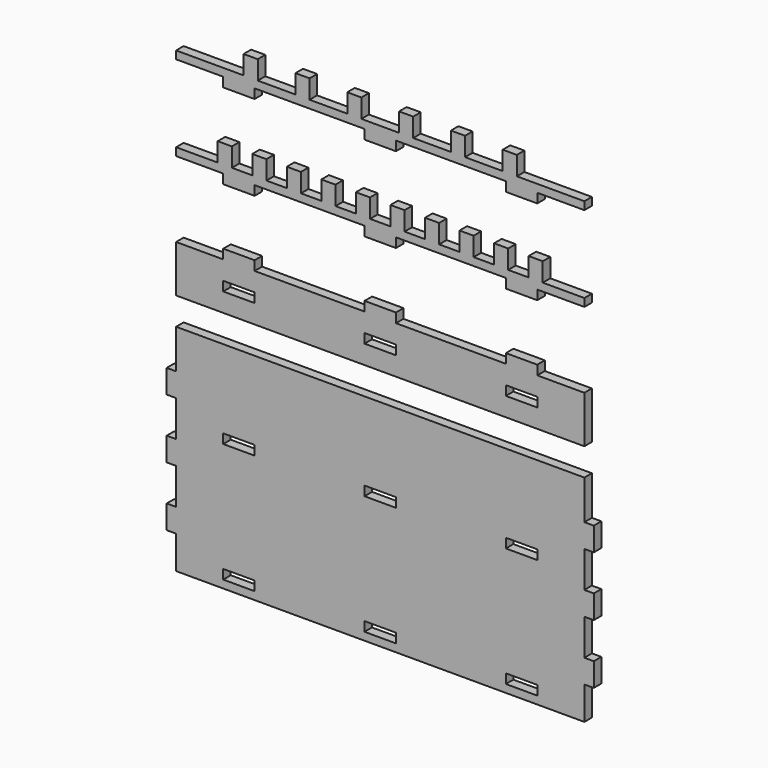
from build123d import *

# Parameters (mm, degrees)
F0_W     = 20
F0_H     = 6
F1_DEPTH = 6
F2_DEPTH = 6
F3_DEPTH = 6
F4_DEPTH = 6


# Not quite as in the source:
# - a feature names something its author has since deleted; it is built from what else it names


with BuildPart() as f1:
    # F0 (on Front) → F1 (new body)
    with BuildSketch(Plane.XZ):
        Polygon((153.699216228, -140.3053558618), (-106.300783772, -140.3053558618), (-106.300783772, -165.3053558618), (-112.300783772, -165.3053558618), (-112.300783772, -180.3053558618), (-106.300783772, -180.3053558618), (-106.300783772, -203.3053558618), (-112.300783772, -203.3053558618), (-112.300783772, -218.3053558618), (-106.300783772, -218.3053558618), (-106.300783772, -241.3053558618), (-112.300783772, -241.3053558618), (-112.300783772, -256.3053558618), (-106.300783772, -256.3053558618), (-106.300783772, -277.3053558618), (153.699216228, -277.3053558618), (153.699216228, -256.3053558618), (159.699216228, -256.3053558618), (159.699216228, -241.3053558618), (153.699216228, -241.3053558618), (153.699216228, -218.3053558618), (159.699216228, -218.3053558618), (159.699216228, -203.3053558618), (153.699216228, -203.3053558618), (153.699216228, -180.3053558618), (159.699216228, -180.3053558618), (159.699216228, -165.3053558618), (153.699216228, -165.3053558618), align=None)
        with Locations((-66.300783772, -269.3053558618)):
            Rectangle(F0_W, F0_H, mode=Mode.SUBTRACT)
        with Locations((-66.300783772, -193.3053558618)):
            Rectangle(F0_W, F0_H, mode=Mode.SUBTRACT)
        with Locations((23.699216228, -193.3053558618)):
            Rectangle(F0_W, F0_H, mode=Mode.SUBTRACT)
        with Locations((23.699216228, -269.3053558618)):
            Rectangle(F0_W, F0_H, mode=Mode.SUBTRACT)
        with Locations((113.699216228, -269.3053558618)):
            Rectangle(F0_W, F0_H, mode=Mode.SUBTRACT)
        with Locations((113.699216228, -193.3053558618)):
            Rectangle(F0_W, F0_H, mode=Mode.SUBTRACT)
    extrude(amount=F1_DEPTH)


with BuildPart() as f2:
    # F0 (on Front) → F2 (new body)
    with BuildSketch(Plane.XZ):
        Polygon((-76.300783772, -92.7685894072), (-106.300783772, -92.7685894072), (-106.300783772, -122.7685894072), (153.699216228, -122.7685894072), (153.699216228, -92.7685894072), (123.699216228, -92.7685894072), (123.699216228, -86.7685894072), (103.699216228, -86.7685894072), (103.699216228, -92.7685894072), (33.699216228, -92.7685894072), (33.699216228, -86.7685894072), (13.699216228, -86.7685894072), (13.699216228, -92.7685894072), (-56.300783772, -92.7685894072), (-56.300783772, -86.7685894072), (-76.300783772, -86.7685894072), align=None)
        with Locations((-66.300783772, -107.7685894072)):
            Rectangle(F0_W, F0_H, mode=Mode.SUBTRACT)
        with Locations((23.699216228, -107.7685894072)):
            Rectangle(F0_W, F0_H, mode=Mode.SUBTRACT)
        with Locations((113.699216228, -107.7685894072)):
            Rectangle(F0_W, F0_H, mode=Mode.SUBTRACT)
    extrude(amount=F2_DEPTH)


with BuildPart() as f3:
    # F0 (on Front) → F3 (new body)
    with BuildSketch(Plane.XZ):
        Polygon((-63.300783772, 26.6136842668), (-63.300783772, 14.6136842668), (-106.300783772, 14.6136842668), (-106.300783772, 9.6136842668), (-76.300783772, 9.6136842668), (-76.300783772, 3.6136842668), (-56.300783772, 3.6136842668), (-56.300783772, 9.6136842668), (13.699216228, 9.6136842668), (13.699216228, 3.6136842668), (33.699216228, 3.6136842668), (33.699216228, 9.6136842668), (103.699216228, 9.6136842668), (103.699216228, 3.6136842668), (123.699216228, 3.6136842668), (123.699216228, 9.6136842668), (153.699216228, 9.6136842668), (153.699216228, 14.6136842668), (134.699216228, 14.6136842668), (110.699216228, 14.6136842668), (110.699216228, 26.6136842668), (101.699216228, 26.6136842668), (101.699216228, 14.6136842668), (77.699216228, 14.6136842668), (77.699216228, 26.6136842668), (68.699216228, 26.6136842668), (68.699216228, 14.6136842668), (44.699216228, 14.6136842668), (44.699216228, 26.6136842668), (35.699216228, 26.6136842668), (35.699216228, 14.6136842668), (11.699216228, 14.6136842668), (11.699216228, 26.6136842668), (2.699216228, 26.6136842668), (2.699216228, 14.6136842668), (-21.300783772, 14.6136842668), (-21.300783772, 26.6136842668), (-30.300783772, 26.6136842668), (-30.300783772, 14.6136842668), (-54.300783772, 14.6136842668), (-54.300783772, 26.6136842668), align=None)
    extrude(amount=F3_DEPTH)


with BuildPart() as f4:
    # F0 (on Front) → F4 (new body)
    with BuildSketch(Plane.XZ):
        Polygon((-79.800783772, -27.6473498154), (-79.800783772, -39.6473498154), (-106.300783772, -39.6473498154), (-106.300783772, -44.6473498154), (-76.300783772, -44.6473498154), (-76.300783772, -50.6473498154), (-56.300783772, -50.6473498154), (-56.300783772, -44.6473498154), (13.699216228, -44.6473498154), (13.699216228, -50.6473498154), (33.699216228, -50.6473498154), (33.699216228, -44.6473498154), (103.699216228, -44.6473498154), (103.699216228, -50.6473498154), (123.699216228, -50.6473498154), (123.699216228, -44.6473498154), (153.699216228, -44.6473498154), (153.699216228, -39.6473498154), (140.199216228, -39.6473498154), (127.199216228, -39.6473498154), (127.199216228, -27.6473498154), (118.199216228, -27.6473498154), (118.199216228, -39.6473498154), (105.199216228, -39.6473498154), (105.199216228, -27.6473498154), (96.199216228, -27.6473498154), (96.199216228, -39.6473498154), (83.199216228, -39.6473498154), (83.199216228, -27.6473498154), (74.199216228, -27.6473498154), (74.199216228, -39.6473498154), (61.199216228, -39.6473498154), (61.199216228, -27.6473498154), (52.199216228, -27.6473498154), (52.199216228, -39.6473498154), (39.199216228, -39.6473498154), (39.199216228, -27.6473498154), (30.199216228, -27.6473498154), (30.199216228, -39.6473498154), (17.199216228, -39.6473498154), (17.199216228, -27.6473498154), (8.199216228, -27.6473498154), (8.199216228, -39.6473498154), (-4.800783772, -39.6473498154), (-4.800783772, -27.6473498154), (-13.800783772, -27.6473498154), (-13.800783772, -39.6473498154), (-26.800783772, -39.6473498154), (-26.800783772, -27.6473498154), (-35.800783772, -27.6473498154), (-35.800783772, -39.6473498154), (-48.800783772, -39.6473498154), (-48.800783772, -27.6473498154), (-57.800783772, -27.6473498154), (-57.800783772, -39.6473498154), (-70.800783772, -39.6473498154), (-70.800783772, -27.6473498154), align=None)
    extrude(amount=F4_DEPTH)


solid = Compound([f1.part, f2.part, f3.part, f4.part])
